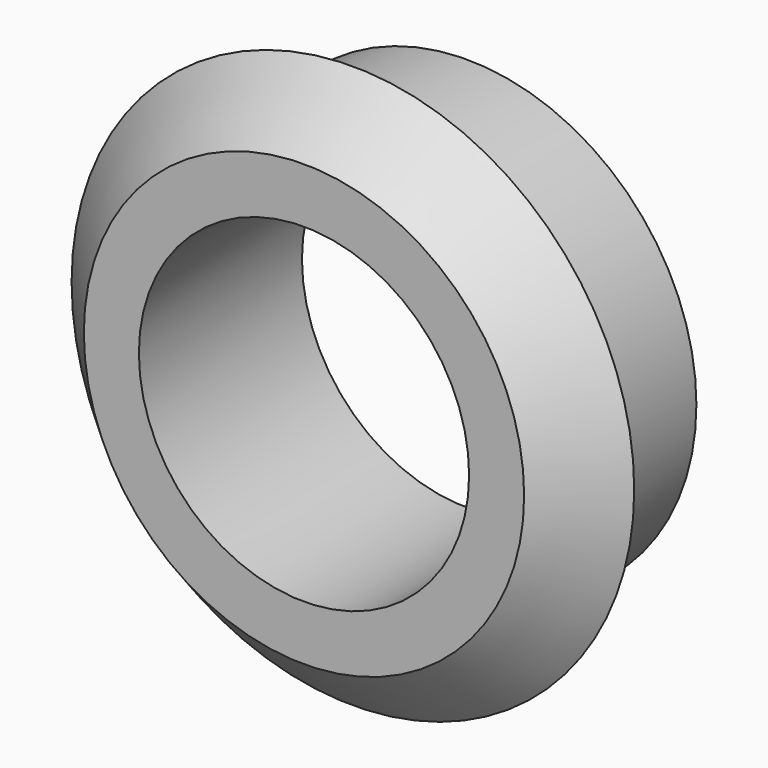
from build123d import *

# Parameters (mm, degrees)
F0_R     = 13.8
F1_DEPTH = 3
F2_R     = 8.1
F3_DEPTH = 25
F2_R_2   = 11.25
F4_DEPTH = 10
F5_SIZE  = 2.99999


# Not quite as in the source:
# - a fillet or chamfer is up to 0.001 mm smaller than in the source, because OpenCascade refuses the exact size


with BuildPart() as f1:
    # F0 (on Front) → F1 (new body)
    with BuildSketch(Plane.XZ):
        Circle(F0_R)
    extrude(amount=F1_DEPTH)

    # F2 (on face) → F3 (cut)
    with BuildSketch(Plane.XZ.offset(3)):
        Circle(F2_R)
    extrude(amount=-F3_DEPTH, mode=Mode.SUBTRACT)

    # F2 (on face) → F4 (join)
    with BuildSketch(Plane.XZ.offset(3)):
        Circle(F2_R_2)
        Circle(F2_R, mode=Mode.SUBTRACT)
    extrude(amount=-F4_DEPTH)

    # F5 (size 3 in the source; OpenCascade refuses exactly that, so slightly less here)
    f5_edges = [f1.edges().sort_by_distance(p)[0] for p in [
        (-13.8, -3, 0),
    ]]
    chamfer(f5_edges, length=F5_SIZE)


solid = f1.part
